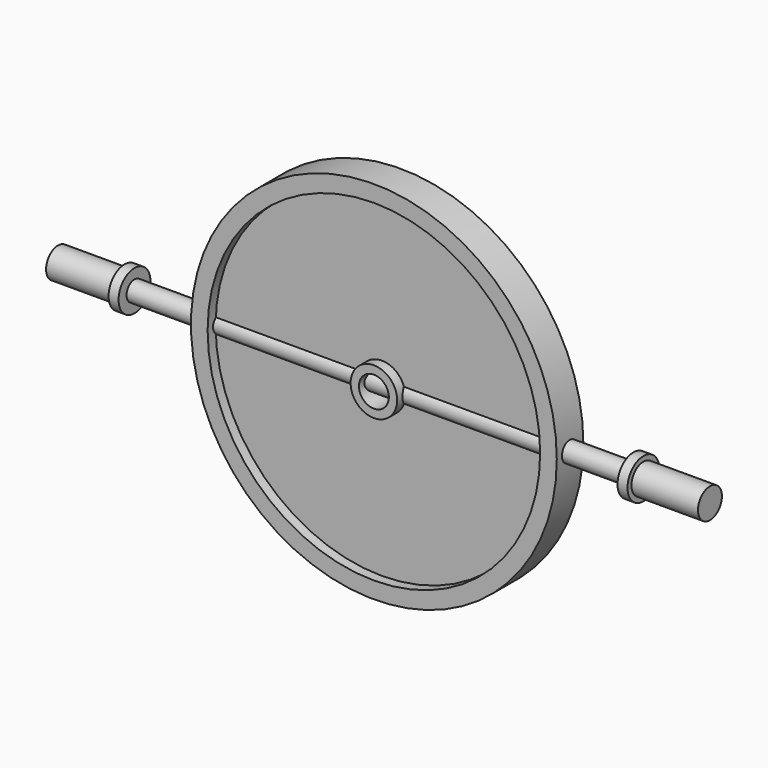
from build123d import *

# Parameters (mm, degrees)
F0_R     = 50
F0_R_2   = 7
F1_DEPTH = 2
F0_R_3   = 55
F2_DEPTH = 5
F0_R_4   = 4.5
F5_DEPTH = 5


with BuildPart() as f1:
    # F0 (on Front) → F1 (new body, symmetric)
    with BuildSketch(Plane.XZ):
        Circle(F0_R)
        Circle(F0_R_2, mode=Mode.SUBTRACT)
    extrude(amount=F1_DEPTH, both=True)

    # F0 (on Front) → F2 (join, symmetric)
    with BuildSketch(Plane.XZ):
        Circle(F0_R_3)
        Circle(F0_R, mode=Mode.SUBTRACT)
    extrude(amount=F2_DEPTH, both=True)

    # F0 (on Front) → F5 (join, symmetric)
    with BuildSketch(Plane.XZ):
        Circle(F0_R_2)
        Circle(F0_R_4, mode=Mode.SUBTRACT)
    extrude(amount=F5_DEPTH, both=True)


with BuildPart() as f4:
    # F3 (on Front) → F4 (revolve)
    with BuildSketch(Plane.XZ):
        Polygon((-98.9746183659, 0), (97.0577100897, 0), (97.0577100897, 4.5), (77.0577100897, 4.5), (77.0577100897, 6), (74.0577100897, 6), (74.0577100897, 3), (-75.9746183659, 3), (-75.9746183659, 6), (-78.9746183659, 6), (-78.9746183659, 4.5), (-98.9746183659, 4.5), align=None)
    revolve(axis=Axis((-0.9584541381, 0, 0), (1, 0, 0)))


solid = Compound([f1.part, f4.part])
